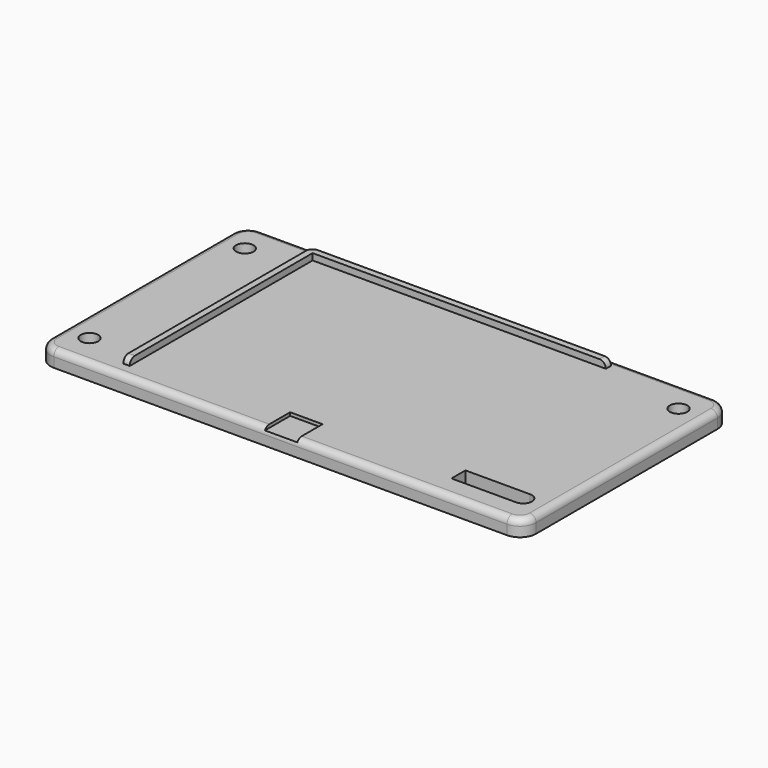
from build123d import *

# Parameters (mm, degrees)
F0_W         = 150
F0_H         = 80
F0_R         = 2.7
F1_DEPTH     = 5
F3_DEPTH     = 2
F4_R         = 5
F5_R         = 1.99999
F6_R         = 2
F7_W         = 10
F7_H         = 10
F8_DEPTH     = 1
F9_T1_DEPTH  = 70
F9_T3_DEPTH  = 140
F9_T5_DEPTH  = 70
F9_T7_DEPTH  = 70
F9_T10_ANGLE = 90
F9_T12_ANGLE = 90
F9_T14_ANGLE = 90
F9_T16_ANGLE = 90


# Not quite as in the source:
# - a fillet or chamfer that OpenCascade refuses, or shapes differently, is made with other operations: its cross-section is extruded or revolved along the edge and cut away or added
# - a fillet or chamfer is up to 0.001 mm smaller than in the source, because OpenCascade refuses the exact size
# - a feature names something its author has since deleted; it is built from what else it names


with BuildPart() as f1:
    # F0 (on Top) → F1 (new body)
    with BuildSketch(Plane.XY):
        Rectangle(F0_W, F0_H)
        with Locations((-67, -30)):
            Circle(F0_R, mode=Mode.SUBTRACT)
        with BuildLine():
            ThreePointArc((67, -27.3), (68.9091883092, -28.0908116908), (69.7, -30))
            ThreePointArc((69.7, -30), (68.9091883092, -31.9091883092), (67, -32.7))
            Line((67, -32.7), (47, -32.7))
            Line((47, -32.7), (47, -27.3))
            Line((47, -27.3), (67, -27.3))
        make_face(mode=Mode.SUBTRACT)
        with Locations((-67, 30)):
            Circle(F0_R, mode=Mode.SUBTRACT)
        with Locations((67, 30)):
            Circle(F0_R, mode=Mode.SUBTRACT)
    extrude(amount=F1_DEPTH)

    # F2 (on face) → F3 (join)
    with BuildSketch(Plane.XY.offset(5)):
        Polygon((-50.3, -35.3), (-50.3, 35.3), (40.3, 35.3), (40.3, 37.3), (-52.3, 37.3), (-52.3, -35.3), align=None)
    extrude(amount=F3_DEPTH)

    # F4
    f4_edges = [f1.edges().sort_by_distance(p)[0] for p in [
        (75, -40, 2.5),
        (-75, -40, 2.5),
        (-75, 40, 2.5),
        (75, 40, 2.5),
    ]]
    fillet(f4_edges, radius=F4_R)

    # F5 (radius 2 in the source; OpenCascade refuses exactly that, so slightly less here)
    f5_edges = [f1.edges().sort_by_distance(p)[0] for p in [
        (-51.3, -35.3, 7),
        (40.3, 36.3, 7),
    ]]
    fillet(f5_edges, radius=F5_R)

    # F6
    f6_edges = [f1.edges().sort_by_distance(p)[0] for p in [
        (-52.3, 37.3, 6),
    ]]
    fillet(f6_edges, radius=F6_R)

    # F7 (on face) → F8 (cut)
    with BuildSketch(Plane.XY.offset(5)):
        with Locations((0, -35)):
            Rectangle(F7_W, F7_H)
    extrude(amount=-F8_DEPTH, mode=Mode.SUBTRACT)

    # F9: fillet of radius 2 on 7 edges, made by hand

    # F9_s2 → F9_t1 (cut)
    with BuildSketch(Plane.XZ.offset(-35)):
        with BuildLine():
            ThreePointArc((-73, 5), (-74.4142135624, 4.4142135624), (-75, 3))
            Line((-75, 3), (-75, 5))
            Line((-75, 5), (-73, 5))
        make_face()
        with BuildLine():
            ThreePointArc((73, 5), (74.4142135624, 4.4142135624), (75, 3))
            Line((75, 3), (75, 5))
            Line((75, 5), (73, 5))
        make_face()
    extrude(amount=F9_T1_DEPTH, mode=Mode.SUBTRACT)

    # F9_s4 → F9_t3 (cut)
    with BuildSketch(Plane.YZ.offset(-70)):
        with BuildLine():
            ThreePointArc((38, 5), (39.4142135624, 4.4142135624), (40, 3))
            Line((40, 3), (40, 5))
            Line((40, 5), (38, 5))
        make_face()
    extrude(amount=F9_T3_DEPTH, mode=Mode.SUBTRACT)

    # F9_s6 → F9_t5 (cut)
    with BuildSketch(Plane.YZ):
        with BuildLine():
            ThreePointArc((-38, 5), (-39.4142135624, 4.4142135624), (-40, 3))
            Line((-40, 3), (-40, 5))
            Line((-40, 5), (-38, 5))
        make_face()
    extrude(amount=F9_T5_DEPTH, mode=Mode.SUBTRACT)

    # F9_s8 → F9_t7 (cut)
    with BuildSketch(Plane.YZ.offset(-70)):
        with BuildLine():
            ThreePointArc((-38, 5), (-39.4142135624, 4.4142135624), (-40, 3))
            Line((-40, 3), (-40, 5))
            Line((-40, 5), (-38, 5))
        make_face()
    extrude(amount=F9_T7_DEPTH, mode=Mode.SUBTRACT)

    # F9_s9 → F9_t10 (revolve, cut)
    with BuildSketch(Plane.XZ.offset(35)):
        with BuildLine():
            ThreePointArc((-73, 5), (-74.4142135624, 4.4142135624), (-75, 3))
            Line((-75, 3), (-75, 5))
            Line((-75, 5), (-73, 5))
        make_face()
    revolve(axis=Axis((-70, -35, 5), (0, 0, 1)), revolution_arc=F9_T10_ANGLE, mode=Mode.SUBTRACT)

    # F9_s11 → F9_t12 (revolve, cut)
    with BuildSketch(Plane.XZ.offset(35)):
        with BuildLine():
            ThreePointArc((73, 5), (74.4142135624, 4.4142135624), (75, 3))
            Line((75, 3), (75, 5))
            Line((75, 5), (73, 5))
        make_face()
    revolve(axis=Axis((70, -35, 5), (0, 0, -1)), revolution_arc=F9_T12_ANGLE, mode=Mode.SUBTRACT)

    # F9_s13 → F9_t14 (revolve, cut)
    with BuildSketch(Plane.YZ.offset(70)):
        with BuildLine():
            ThreePointArc((38, 5), (39.4142135624, 4.4142135624), (40, 3))
            Line((40, 3), (40, 5))
            Line((40, 5), (38, 5))
        make_face()
    revolve(axis=Axis((70, 35, 5), (0, 0, -1)), revolution_arc=F9_T14_ANGLE, mode=Mode.SUBTRACT)

    # F9_s15 → F9_t16 (revolve, cut)
    with BuildSketch(Plane.YZ.offset(-70)):
        with BuildLine():
            ThreePointArc((38, 5), (39.4142135624, 4.4142135624), (40, 3))
            Line((40, 3), (40, 5))
            Line((40, 5), (38, 5))
        make_face()
    revolve(axis=Axis((-70, 35, 5), (0, 0, 1)), revolution_arc=F9_T16_ANGLE, mode=Mode.SUBTRACT)


solid = f1.part
